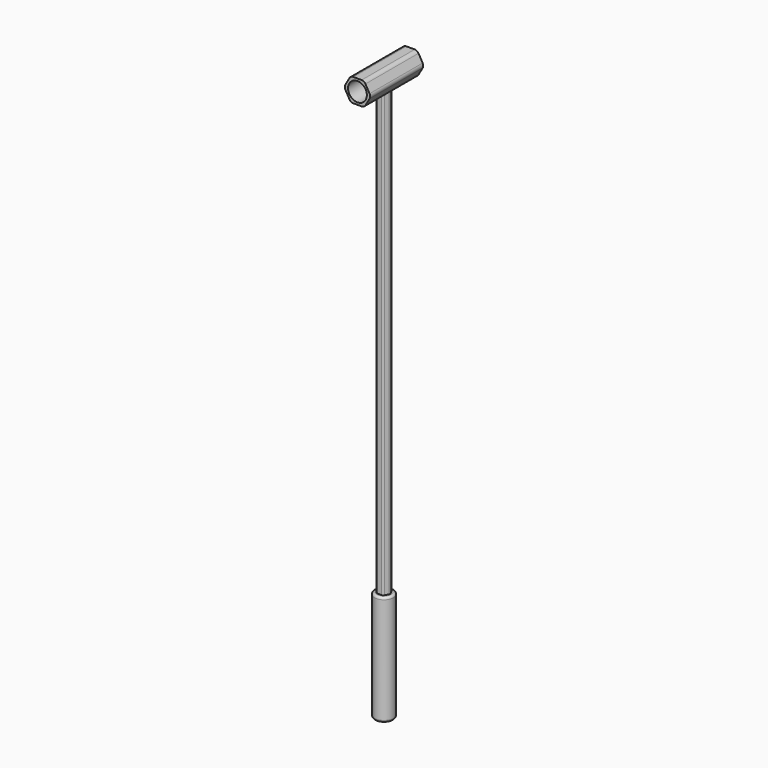
from build123d import *

# Parameters (mm, degrees)
F0_R         = 4.25
F1_DEPTH     = 30
F3_DEPTH     = 200
F4_R         = 4.25
F5_DEPTH     = 50
F6_T1_DEPTH  = 35.7735026919
F6_T6_DEPTH  = 35.7735026919
F6_T12_DEPTH = 35.7735026919
F6_T18_DEPTH = 35.7735026919
F6_T24_DEPTH = 35.7735026919
F6_T30_DEPTH = 35.7735026919
F6_T36_DEPTH = 35.7735026919
F7_R         = 1
F8_R         = 1


# Not quite as in the source:
# - a fillet or chamfer that OpenCascade refuses, or shapes differently, is made with other operations: its cross-section is extruded or revolved along the edge and cut away or added


with BuildPart() as f1:
    # F0 (on Front) → F1 (new body)
    with BuildSketch(Plane.XZ):
        Polygon((3.0310889132, 5.25), (-3.0310889132, 5.25), (-6.0621778265, 0), (-3.0310889132, -5.25), (3.0310889132, -5.25), (6.0621778265, 0), align=None)
        Circle(F0_R, mode=Mode.SUBTRACT)
    extrude(amount=F1_DEPTH)

    # F2 (on face) → F3 (join)
    with BuildSketch(Plane(origin=(0, 0, -5.25), x_dir=(1, 0, 0), z_dir=(0, 0, -1))):
        Polygon((-1.443375673, 12.5), (0, 12.5), (1.443375673, 12.5), (2.8867513459, 15), (1.443375673, 17.5), (-1.443375673, 17.5), (-2.8867513459, 15), align=None)
    extrude(amount=F3_DEPTH)

    # F4 (on face) → F5 (join)
    with BuildSketch(Plane(origin=(0, 0, -205.25), x_dir=(1, 0, 0), z_dir=(0, 0, -1))):
        with Locations((0, 15)):
            Circle(F4_R)
        Polygon((-1.443375673, 12.5), (-2.8867513459, 15), (-1.443375673, 17.5), (1.443375673, 17.5), (2.8867513459, 15), (1.443375673, 12.5), align=None, mode=Mode.SUBTRACT)
        Polygon((-1.443375673, 17.5), (-2.8867513459, 15), (-1.443375673, 12.5), (1.443375673, 12.5), (2.8867513459, 15), (1.443375673, 17.5), align=None)
    extrude(amount=F5_DEPTH)

    # F6: fillet of radius 2 on 6 edges, made by hand

    # F6_s2 → F6_t1 (cut)
    with BuildSketch(Plane.XZ.offset(-2.8867513459)):
        with BuildLine():
            ThreePointArc((5.4848275573, -1), (5.7527767497, 0), (5.4848275573, 1))
            Line((5.4848275573, 1), (6.0621778265, 0))
            Line((6.0621778265, 0), (5.4848275573, -1))
        make_face()
        with BuildLine():
            ThreePointArc((1.8763883749, 5.25), (2.8763883749, 4.9820508076), (3.6084391824, 4.25))
            Line((3.6084391824, 4.25), (3.0310889132, 5.25))
            Line((3.0310889132, 5.25), (1.8763883749, 5.25))
        make_face()
        with BuildLine():
            ThreePointArc((-3.6084391824, 4.25), (-2.8763883749, 4.9820508076), (-1.8763883749, 5.25))
            Line((-1.8763883749, 5.25), (-3.0310889132, 5.25))
            Line((-3.0310889132, 5.25), (-3.6084391824, 4.25))
        make_face()
        with BuildLine():
            ThreePointArc((-5.4848275573, -1), (-5.7527767497, 0), (-5.4848275573, 1))
            Line((-5.4848275573, 1), (-6.0621778265, 0))
            Line((-6.0621778265, 0), (-5.4848275573, -1))
        make_face()
    extrude(amount=F6_T1_DEPTH, mode=Mode.SUBTRACT)


with BuildPart() as f6_tool4:
    # F6_s5 → F6_t6 (new body)
    with BuildSketch(Plane.XZ.offset(-2.8867513459)):
        with BuildLine():
            ThreePointArc((1.8763883749, -5.25), (2.8763883749, -4.9820508076), (3.6084391824, -4.25))
            Line((3.6084391824, -4.25), (3.0310889132, -5.25))
            Line((3.0310889132, -5.25), (1.8763883749, -5.25))
        make_face()
    extrude(amount=F6_T6_DEPTH)

    split(bisect_by=Plane(origin=(-4.3301270189, -2.5, 0), x_dir=(0, 0, 1), z_dir=(0.8660254038, 0.5, 0)), keep=Keep.TOP)

    split(bisect_by=Plane(origin=(8.6602540378, -5, 0), x_dir=(0, 0, 1), z_dir=(-0.8660254038, 0.5, 0)), keep=Keep.TOP)


with BuildPart() as f1_1:
    add(f1.part)

    # F6_t3: cut F6_tool4
    add(f6_tool4.part, mode=Mode.SUBTRACT)


with BuildPart() as f6_tool10:
    # F6_s11 → F6_t12 (new body)
    with BuildSketch(Plane.XZ.offset(-2.8867513459)):
        with BuildLine():
            ThreePointArc((1.8763883749, -5.25), (2.8763883749, -4.9820508076), (3.6084391824, -4.25))
            Line((3.6084391824, -4.25), (3.0310889132, -5.25))
            Line((3.0310889132, -5.25), (1.8763883749, -5.25))
        make_face()
    extrude(amount=F6_T12_DEPTH)

    split(bisect_by=Plane(origin=(-4.3301270189, -2.5, 0), x_dir=(0, 0, 1), z_dir=(0.8660254038, 0.5, 0)), keep=Keep.TOP)

    split(bisect_by=Plane(origin=(8.6602540378, -5, 0), x_dir=(0, 0, 1), z_dir=(0.8660254038, -0.5, 0)), keep=Keep.TOP)


with BuildPart() as f1_2:
    add(f1_1.part)

    # F6_t9: cut F6_tool10
    add(f6_tool10.part, mode=Mode.SUBTRACT)


with BuildPart() as f6_tool16:
    # F6_s17 → F6_t18 (new body)
    with BuildSketch(Plane.XZ.offset(-2.8867513459)):
        with BuildLine():
            ThreePointArc((1.8763883749, -5.25), (2.8763883749, -4.9820508076), (3.6084391824, -4.25))
            Line((3.6084391824, -4.25), (3.0310889132, -5.25))
            Line((3.0310889132, -5.25), (1.8763883749, -5.25))
        make_face()
    extrude(amount=F6_T18_DEPTH)

    split(bisect_by=Plane(origin=(-4.3301270189, -2.5, 0), x_dir=(0, 0, 1), z_dir=(-0.8660254038, -0.5, 0)), keep=Keep.TOP)

    split(bisect_by=Plane(origin=(8.6602540378, -5, 0), x_dir=(0, 0, 1), z_dir=(0.8660254038, -0.5, 0)), keep=Keep.TOP)


with BuildPart() as f1_3:
    add(f1_2.part)

    # F6_t15: cut F6_tool16
    add(f6_tool16.part, mode=Mode.SUBTRACT)


with BuildPart() as f6_tool22:
    # F6_s23 → F6_t24 (new body)
    with BuildSketch(Plane.XZ.offset(-2.8867513459)):
        with BuildLine():
            ThreePointArc((-1.8763883749, -5.25), (-2.8763883749, -4.9820508076), (-3.6084391824, -4.25))
            Line((-3.6084391824, -4.25), (-3.0310889132, -5.25))
            Line((-3.0310889132, -5.25), (-1.8763883749, -5.25))
        make_face()
    extrude(amount=F6_T24_DEPTH)

    split(bisect_by=Plane(origin=(-8.6602540378, -5, 0), x_dir=(0, 0, 1), z_dir=(0.8660254038, 0.5, 0)), keep=Keep.TOP)

    split(bisect_by=Plane(origin=(4.3301270189, -2.5, 0), x_dir=(0, 0, 1), z_dir=(-0.8660254038, 0.5, 0)), keep=Keep.TOP)


with BuildPart() as f1_4:
    add(f1_3.part)

    # F6_t21: cut F6_tool22
    add(f6_tool22.part, mode=Mode.SUBTRACT)


with BuildPart() as f6_tool28:
    # F6_s29 → F6_t30 (new body)
    with BuildSketch(Plane.XZ.offset(-2.8867513459)):
        with BuildLine():
            ThreePointArc((-1.8763883749, -5.25), (-2.8763883749, -4.9820508076), (-3.6084391824, -4.25))
            Line((-3.6084391824, -4.25), (-3.0310889132, -5.25))
            Line((-3.0310889132, -5.25), (-1.8763883749, -5.25))
        make_face()
    extrude(amount=F6_T30_DEPTH)

    split(bisect_by=Plane(origin=(-8.6602540378, -5, 0), x_dir=(0, 0, 1), z_dir=(-0.8660254038, -0.5, 0)), keep=Keep.TOP)

    split(bisect_by=Plane(origin=(4.3301270189, -2.5, 0), x_dir=(0, 0, 1), z_dir=(-0.8660254038, 0.5, 0)), keep=Keep.TOP)


with BuildPart() as f1_5:
    add(f1_4.part)

    # F6_t27: cut F6_tool28
    add(f6_tool28.part, mode=Mode.SUBTRACT)


with BuildPart() as f6_tool34:
    # F6_s35 → F6_t36 (new body)
    with BuildSketch(Plane.XZ.offset(-2.8867513459)):
        with BuildLine():
            ThreePointArc((-1.8763883749, -5.25), (-2.8763883749, -4.9820508076), (-3.6084391824, -4.25))
            Line((-3.6084391824, -4.25), (-3.0310889132, -5.25))
            Line((-3.0310889132, -5.25), (-1.8763883749, -5.25))
        make_face()
    extrude(amount=F6_T36_DEPTH)

    split(bisect_by=Plane(origin=(-8.6602540378, -5, 0), x_dir=(0, 0, 1), z_dir=(-0.8660254038, -0.5, 0)), keep=Keep.TOP)

    split(bisect_by=Plane(origin=(4.3301270189, -2.5, 0), x_dir=(0, 0, 1), z_dir=(0.8660254038, -0.5, 0)), keep=Keep.TOP)


with BuildPart() as f1_6:
    add(f1_5.part)

    # F6_t33: cut F6_tool34
    add(f6_tool34.part, mode=Mode.SUBTRACT)

    # F7
    f7_edges = [f1_6.edges().sort_by_distance(p)[0] for p in [
        (-1.443376, -17.5, -105.25),
        (1.443376, -17.5, -105.25),
        (-2.886751, -15, -105.113013),
        (-1.443376, -12.5, -105.25),
        (2.886751, -15, -105.113013),
        (1.443376, -12.5, -105.25),
    ]]
    fillet(f7_edges, radius=F7_R)

    # F8
    f8_edges = [f1_6.edges().sort_by_distance(p)[0] for p in [
        (-4.25, -15, -255.25),
        (-4.25, -15, -205.25),
    ]]
    fillet(f8_edges, radius=F8_R)


solid = f1_6.part
